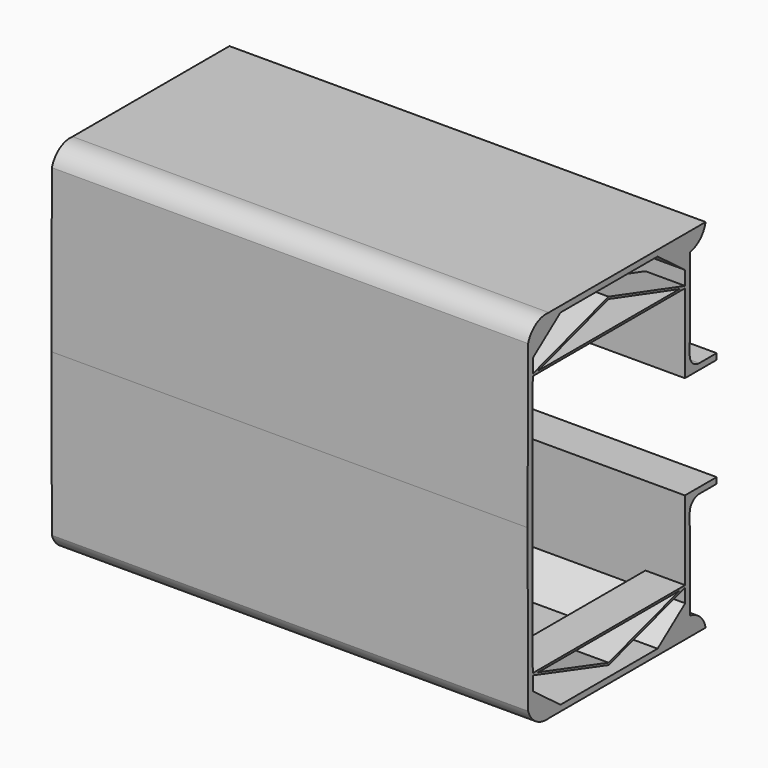
from build123d import *

# Parameters (mm, degrees)
F1_DEPTH = 60
F3_DEPTH = 10


# Not quite as in the source:
# - a feature names something its author has since deleted; it is built from what else it names


with BuildPart() as f1:
    # F0 (on Right) → F1 (new body)
    with BuildSketch(Plane.YZ):
        with BuildLine():
            Line((24.139301102, -43.2624049591), (15.4307844338, -49.7964277864))
            Line((15.4307844338, -49.7964277864), (-15.1525954085, -49.7964277864))
            Line((-15.1525954085, -49.7964277864), (-23.8611120767, -43.2624049591))
            Line((-23.8611120767, -43.2624049591), (-24.0144912707, -6.2964277864))
            Line((-24.0144912707, -6.2964277864), (-25.5145041825, -6.2964277864))
            Line((-25.5145041825, -6.2964277864), (-25.3453201973, -47.0715236276))
            ThreePointArc((-25.3453201973, -47.0715236276), (-22.8573335388, -50.3682627369), (-18.8327744315, -51.2964277864))
            Line((-18.8327744315, -51.2964277864), (30.5735625925, -51.2964277864))
            ThreePointArc((30.5735625925, -51.2964277864), (28.8360021374, -48.2011592055), (25.6532847593, -46.6294995689))
            Line((25.6532847593, -46.6294995689), (25.5585974487, -23.8088752761))
            ThreePointArc((25.5585974487, -23.8088752761), (26.432854985, -21.6795128694), (28.5585716253, -20.7964277864))
            Line((28.5585716253, -20.7964277864), (34.0398614944, -20.7964277864))
            Line((34.0398614944, -20.7964277864), (34.0398614944, -19.2964277864))
            Line((34.0398614944, -19.2964277864), (24.0398614944, -19.2964277864))
            Line((24.0398614944, -19.2964277864), (24.139301102, -43.2624049591))
        make_face()
    extrude(amount=F1_DEPTH)

    # F2 (on face) → F3 (join)
    with BuildSketch(Plane.YZ.offset(60)):
        Polygon((24.1226036063, -39.2381352516), (-23.8778095724, -39.2381352516), (-23.8757047067, -39.7454297089), (-0.0007817785, -47.1604929972), (24.1247084719, -39.7454297089), align=None)
        Polygon((0, -46.6294995689), (-22.1652372944, -39.7454297089), (22.3978614654, -39.7454297089), align=None, mode=Mode.SUBTRACT)
    extrude(amount=-F3_DEPTH)

    # F4: F1 across plane


with BuildPart() as f1_1:
    add(f1.part)
    add(f1.part.mirror(Plane.YZ))

    # F5: F1 across face


with BuildPart() as f1_2:
    add(f1_1.part)
    add(f1_1.part.mirror(Plane(origin=(0, -24.7644977266, -6.2964277864), x_dir=(1, 0, 0), z_dir=(0, 0, 1))))


solid = f1_2.part
